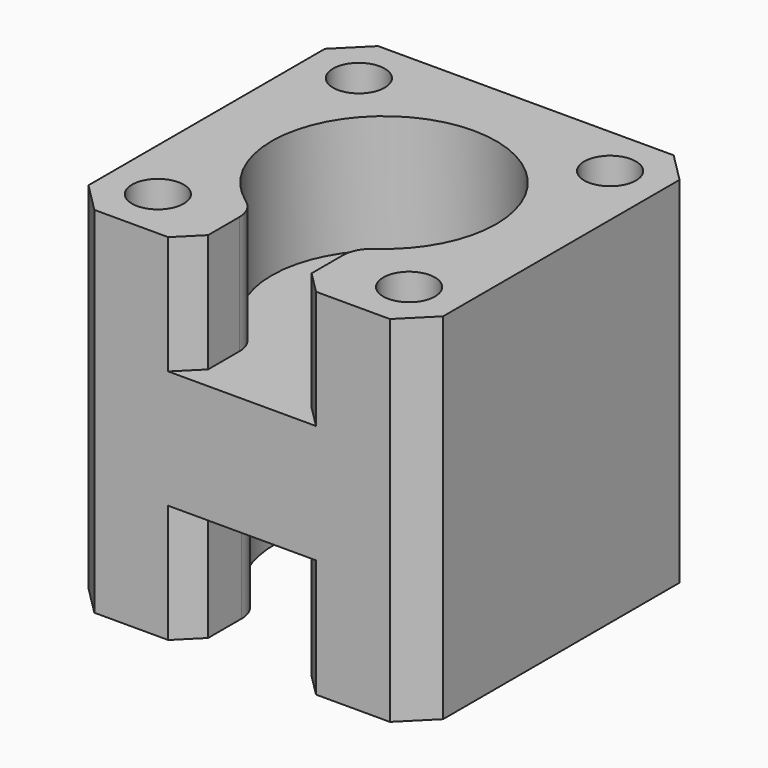
from build123d import *

# Parameters (mm, degrees)
F0_W      = 24
F0_H      = 24
F0_R      = 2.6
F1_DEPTH  = 24
F2_SIZE   = 2
F4_DEPTH  = 8
F5_R      = 2
F7_DEPTH  = 8
F8_R      = 2
F9_SIZE   = 1.5
F10_R     = 1.75
F11_DEPTH = 25


with BuildPart() as f1:
    # F0 (on Top) → F1 (new body)
    with BuildSketch(Plane.XY):
        Rectangle(F0_W, F0_H)
        Circle(F0_R, mode=Mode.SUBTRACT)
    extrude(amount=F1_DEPTH)

    # F2
    f2_edges = [f1.edges().sort_by_distance(p)[0] for p in [
        (-12, -12, 12),
        (12, -12, 12),
        (-12, 12, 12),
        (12, 12, 12),
    ]]
    chamfer(f2_edges, length=F2_SIZE)

    # F3 (on Top) → F4 (cut)
    with BuildSketch(Plane.XY):
        with BuildLine():
            ThreePointArc((3.5, -6.5611658181), (6.3767557079, -3.8256873283), (7.4363228072, 0))
            ThreePointArc((7.4363228072, 0), (-3.8256873283, 6.3767557079), (-3.5, -6.5611658181))
            Line((-3.5, -6.5611658181), (-3.5, -3))
            Line((-3.5, -3), (3.5, -3))
            Line((3.5, -3), (3.5, -6.5611658181))
        make_face()
        with BuildLine():
            Line((-3.5, -3), (-3.5, -6.5611658181))
            ThreePointArc((-3.5, -6.5611658181), (0, -7.4363228072), (3.5, -6.5611658181))
            Line((3.5, -6.5611658181), (3.5, -3))
            Line((3.5, -3), (-3.5, -3))
        make_face()
        with BuildLine():
            ThreePointArc((3.5, -6.5611658181), (0, -7.4363228072), (-3.5, -6.5611658181))
            Line((-3.5, -6.5611658181), (-3.5, -13))
            Line((-3.5, -13), (3.5, -13))
            Line((3.5, -13), (3.5, -6.5611658181))
        make_face()
    extrude(amount=F4_DEPTH, mode=Mode.SUBTRACT)

    # F5
    f5_edges = [f1.edges().sort_by_distance(p)[0] for p in [
        (-3.5, -6.561166, 4),
        (3.5, -6.561166, 4),
    ]]
    fillet(f5_edges, radius=F5_R)

    # F6 (on face) → F7 (cut)
    with BuildSketch(Plane.XY.offset(24)):
        with BuildLine():
            ThreePointArc((3.5, -6.7461099902), (6.4946131525, -3.9471508712), (7.6, 0))
            ThreePointArc((7.6, 0), (-3.9471508712, 6.4946131525), (-3.5, -6.7461099902))
            Line((-3.5, -6.7461099902), (-3.5, -4.0145893581))
            Line((-3.5, -4.0145893581), (3.5, -4.0145893581))
            Line((3.5, -4.0145893581), (3.5, -6.7461099902))
        make_face()
        with BuildLine():
            Line((-3.5, -4.0145893581), (-3.5, -6.7461099902))
            ThreePointArc((-3.5, -6.7461099902), (0, -7.6), (3.5, -6.7461099902))
            Line((3.5, -6.7461099902), (3.5, -4.0145893581))
            Line((3.5, -4.0145893581), (-3.5, -4.0145893581))
        make_face()
        with BuildLine():
            ThreePointArc((3.5, -6.7461099902), (0, -7.6), (-3.5, -6.7461099902))
            Line((-3.5, -6.7461099902), (-3.5, -12))
            Line((-3.5, -12), (3.5, -12))
            Line((3.5, -12), (3.5, -6.7461099902))
        make_face()
    extrude(amount=-F7_DEPTH, mode=Mode.SUBTRACT)

    # F8
    f8_edges = [f1.edges().sort_by_distance(p)[0] for p in [
        (3.5, -6.74611, 20),
        (-3.5, -6.74611, 20),
    ]]
    fillet(f8_edges, radius=F8_R)

    # F9
    f9_edges = [f1.edges().sort_by_distance(p)[0] for p in [
        (3.5, -12, 20),
        (-3.5, -12, 20),
        (3.5, -12, 4),
        (-3.5, -12, 4),
    ]]
    chamfer(f9_edges, length=F9_SIZE)

    # F10 (on Top) → F11 (cut)
    with BuildSketch(Plane.XY):
        with Locations((-8.5, -8.5)):
            Circle(F10_R)
        with Locations((8.5, -8.5)):
            Circle(F10_R)
        with Locations((8.5, 8.5)):
            Circle(F10_R)
        with Locations((-8.5, 8.5)):
            Circle(F10_R)
    extrude(amount=F11_DEPTH, mode=Mode.SUBTRACT)


solid = f1.part
